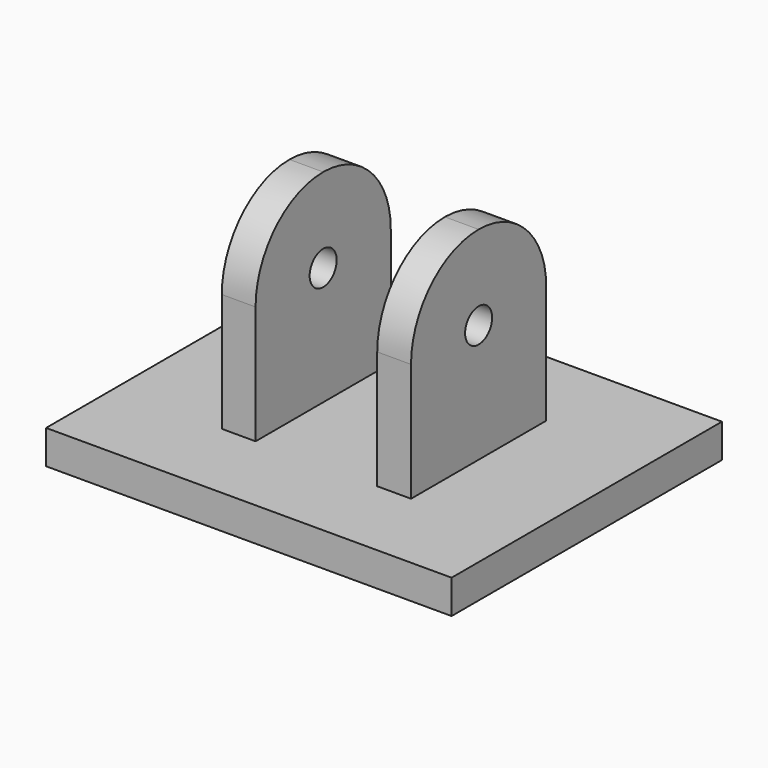
from build123d import *

# Parameters (mm, degrees)
F0_W     = 60
F0_H     = 50
F1_DEPTH = 5
F2_W     = 5
F2_H     = 25
F3_DEPTH = 30
F4_R     = 12.49999
F5_R     = 2.5
F6_DEPTH = 50


# Not quite as in the source:
# - a fillet or chamfer is up to 0.001 mm smaller than in the source, because OpenCascade refuses the exact size


with BuildPart() as f1:
    # F0 (on Top) → F1 (new body)
    with BuildSketch(Plane.XY):
        Rectangle(F0_W, F0_H)
    extrude(amount=F1_DEPTH)

    # F2 (on face) → F3 (join)
    with BuildSketch(Plane.XY.offset(5)):
        with Locations((-11.5, 0)):
            Rectangle(F2_W, F2_H)
        with Locations((11.5, 0)):
            Rectangle(F2_W, F2_H)
    extrude(amount=F3_DEPTH)

    # F4 (radius 12.5 in the source; OpenCascade refuses exactly that, so slightly less here)
    f4_edges = [f1.edges().sort_by_distance(p)[0] for p in [
        (-11.5, -12.5, 35),
        (-11.5, 12.5, 35),
        (11.5, 12.5, 35),
        (11.5, -12.5, 35),
    ]]
    fillet(f4_edges, radius=F4_R)

    # F5 (on face) → F6 (cut)
    with BuildSketch(Plane(origin=(-14, 0, 0), x_dir=(0, -1, 0), z_dir=(-1, 0, 0))):
        with Locations((0, 22.5)):
            Circle(F5_R)
    extrude(amount=-F6_DEPTH, mode=Mode.SUBTRACT)


solid = f1.part
